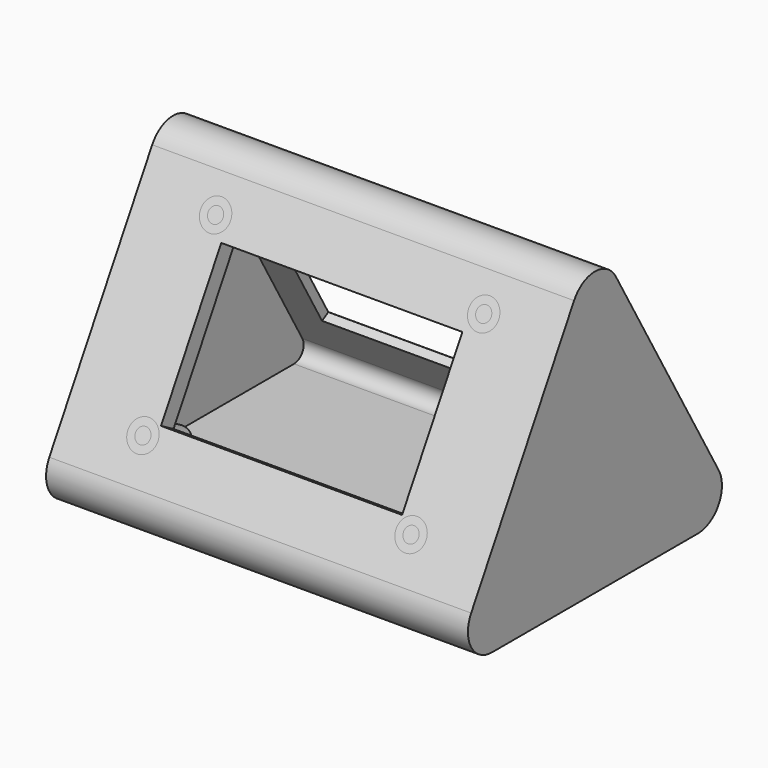
from build123d import *

# Parameters (mm, degrees)
F1_DEPTH  = 35
F2_DEPTH  = 32
F3_R      = 5
F4_R      = 2
F5_W      = 40
F5_H      = 25
F6_DEPTH  = 3
F5_R      = 2.5
F5_R_2    = 1.25
F7_DEPTH  = 8
F8_W      = 52
F8_H      = 29
F9_DEPTH  = 3
F8_W_2    = 60
F8_H_2    = 35
F10_DEPTH = 1.5
F11_R     = 5
F12_DEPTH = 3
F13_D     = 2
F13_DEPTH = 3
F13_TIP   = 0.600860619


with BuildPart() as f1:
    # F0 (on Right) → F1 (new body, symmetric)
    with BuildSketch(Plane.YZ):
        Polygon((-60, 0), (0, 0), (-30, 51.9615242271), align=None)
        Polygon((-5.1961524227, 3), (-54.8038475773, 3), (-30, 45.9615242271), align=None, mode=Mode.SUBTRACT)
        Polygon((-30, 45.9615242271), (-54.8038475773, 3), (-5.1961524227, 3), align=None)
    extrude(amount=F1_DEPTH, both=True)

    # F0 (on Right) → F2 (cut, symmetric)
    with BuildSketch(Plane.YZ):
        Polygon((-30, 45.9615242271), (-54.8038475773, 3), (-5.1961524227, 3), align=None)
    extrude(amount=F2_DEPTH, both=True, mode=Mode.SUBTRACT)

    # F3
    f3_edges = [f1.edges().sort_by_distance(p)[0] for p in [
        (0, -30, 51.961524),
        (0, -60, 0),
        (0, 0, 0),
    ]]
    fillet(f3_edges, radius=F3_R)

    # F4
    f4_edges = [f1.edges().sort_by_distance(p)[0] for p in [
        (0, -30, 45.961524),
        (0, -5.196152, 3),
        (0, -54.803848, 3),
    ]]
    fillet(f4_edges, radius=F4_R)

    # F5 (on face) → F6 (cut)
    with BuildSketch(Plane(origin=(0, -45, 25.9807621135), x_dir=(1, 0, 0), z_dir=(0, -0.8660254038, 0.5))):
        with Locations((0, -0.0002540378)):
            Rectangle(F5_W, F5_H)
    extrude(amount=-F6_DEPTH, mode=Mode.SUBTRACT)

    # F5 (on face) → F7 (join)
    with BuildSketch(Plane(origin=(0, -45, 25.9807621135), x_dir=(1, 0, 0), z_dir=(0, -0.8660254038, 0.5))):
        with Locations((-22.1997145563, 15.6450960785)):
            Circle(F5_R)
        with Locations((-22.1997145563, 15.6450960785)):
            Circle(F5_R_2, mode=Mode.SUBTRACT)
        with Locations((22.287291775, 15.6450960785)):
            Circle(F5_R)
        with Locations((22.287291775, 15.6450960785)):
            Circle(F5_R_2, mode=Mode.SUBTRACT)
        with Locations((22.287291775, -14.4981121665)):
            Circle(F5_R)
        with Locations((22.287291775, -14.4981121665)):
            Circle(F5_R_2, mode=Mode.SUBTRACT)
        with Locations((-22.1997145563, -14.4981121665)):
            Circle(F5_R)
        with Locations((-22.1997145563, -14.4981121665)):
            Circle(F5_R_2, mode=Mode.SUBTRACT)
    extrude(amount=-F7_DEPTH)

    # F8 (on face) → F9 (cut)
    with BuildSketch(Plane(origin=(0, 0, 0), x_dir=(-1, 0, 0), z_dir=(0, 0.8660254038, 0.5))):
        with Locations((0, 30.0002540378)):
            Rectangle(F8_W, F8_H)
    extrude(amount=-F9_DEPTH, mode=Mode.SUBTRACT)

    # F8 (on face) → F10 (cut)
    with BuildSketch(Plane(origin=(0, 0, 0), x_dir=(-1, 0, 0), z_dir=(0, 0.8660254038, 0.5))):
        with Locations((0, 30.0002540378)):
            Rectangle(F8_W_2, F8_H_2)
        with Locations((0, 30.0002540378)):
            Rectangle(F8_W, F8_H, mode=Mode.SUBTRACT)
    extrude(amount=-F10_DEPTH, mode=Mode.SUBTRACT)

    # F11 (on face) → F12 (cut, through all)
    with BuildSketch(Plane(origin=(0, 0, 0), x_dir=(1, 0, 0), z_dir=(0, 0, -1))):
        with Locations((0, 41.3397459622)):
            Circle(F11_R)
    extrude(amount=-F12_DEPTH, mode=Mode.SUBTRACT)

    # F13
    with Locations(Plane(origin=(0, 0, 0), x_dir=(-1, 0, 0), z_dir=(0, 0.8660254038, 0.5))):
        with Locations((-28, 30.0002540378), (28, 30.0002540378)):
            Hole(F13_D / 2, depth=F13_DEPTH)
            with Locations((0, 0, -(F13_DEPTH + F13_TIP / 2))):  # 118° drill point
                Cone(0, F13_D / 2, F13_TIP, mode=Mode.SUBTRACT)


solid = f1.part
